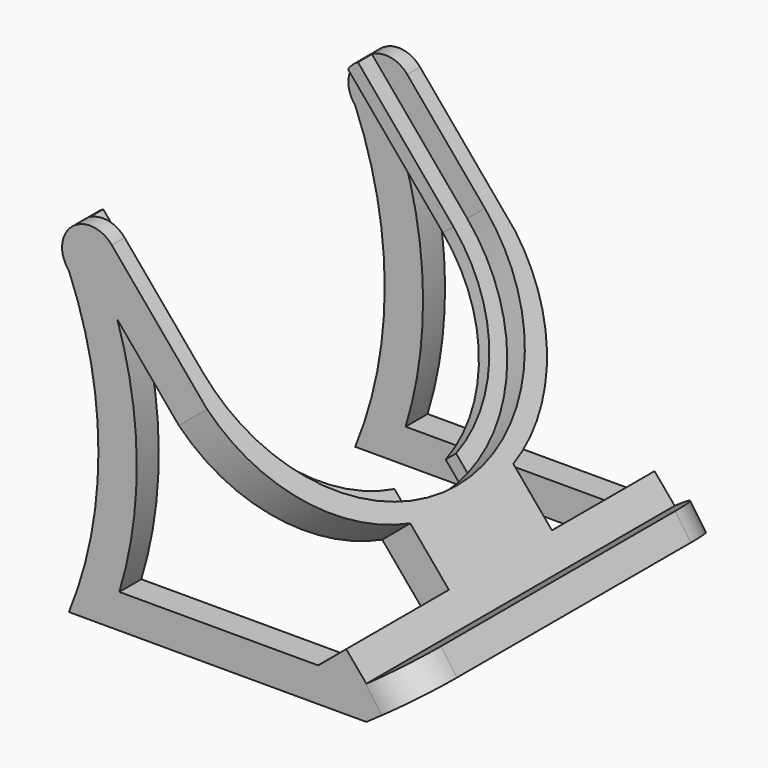
from build123d import *

# Parameters (mm, degrees)
F1_DEPTH  = 53.34
F2_W      = 4.826
F2_H      = 32.1946403572
F3_DEPTH  = 6.35
F5_DEPTH  = 106.68
F7_W      = 91.44
F7_H      = 183.6228075896
F8_DEPTH  = 58.928
F9_DEPTH  = 25.4
F10_R     = 12.8774151417
F11_DEPTH = 10.16
F13_DEPTH = 25.4
F15_DEPTH = 3.81


# Not quite as in the source:
# - a feature names something its author has since deleted; it is built from what else it names


with BuildPart() as f1:
    # F0 (on Front) → F1 (new body, symmetric)
    with BuildSketch(Plane.XZ):
        with BuildLine():
            ThreePointArc((-26.4580316219, 31.2050478526), (-18.2875299748, -10.3937397156), (-26.4580316219, -51.9925272838))
            Line((-26.4580316219, -51.9925272838), (55.8778569108, -51.9925272838))
            Line((55.8778569108, -51.9925272838), (70.650836429, -41.6293909539))
            Line((70.650836429, -41.6293909539), (66.2748063527, -35.3912212887))
            Line((66.2748063527, -35.3912212887), (55.8778569108, -42.6846047493))
            Line((55.8778569108, -42.6846047493), (-14.5902915946, 41.2960643955))
            ThreePointArc((-14.5902915946, 41.2960643955), (-25.6027276184, 42.2233043466), (-26.4580316219, 31.2050478526))
        make_face()
    extrude(amount=F1_DEPTH, both=True)

    # F2 (on face) → F3 (cut)
    with BuildSketch(Plane(origin=(11.772407622, 0, 9.8782228937), x_dir=(0, 1, 0), z_dir=(0.7660444431, 0, 0.6427876097))):
        with BuildLine():
            ThreePointArc((-44.069, 28.7653259742), (-47.673235573, 18.4461288519), (-48.895, 7.584101647))
            Line((-48.895, 7.584101647), (-44.069, 7.584101647))
            Line((-44.069, 7.584101647), (-44.069, 28.7653259742))
        make_face()
        with BuildLine():
            ThreePointArc((44.069, 28.7653259742), (47.673235573, 18.4461288519), (48.895, 7.584101647))
            Line((48.895, 7.584101647), (48.895, 41.0130793115))
            Line((48.895, 41.0130793115), (44.069, 41.0130793115))
            Line((44.069, 41.0130793115), (44.069, 28.7653259742))
        make_face()
        with BuildLine():
            Line((-44.069, 41.0130793115), (-35.6822711903, 41.0130793115))
            ThreePointArc((-35.6822711903, 41.0130793115), (-19.4449371571, 52.4462844288), (0, 56.479101647))
            Line((0, 56.479101647), (0, 73.2077196687))
            Line((0, 73.2077196687), (-44.069, 73.2077196687))
            Line((-44.069, 73.2077196687), (-44.069, 41.0130793115))
        make_face()
        with Locations((-46.482, 57.1103994901)):
            Rectangle(F2_W, F2_H)
        with BuildLine():
            ThreePointArc((0, 56.479101647), (-19.4449371571, 52.4462844288), (-35.6822711903, 41.0130793115))
            Line((-35.6822711903, 41.0130793115), (-28.7155047544, 41.0130793115))
            ThreePointArc((-28.7155047544, 41.0130793115), (-15.3116809054, 48.9075718407), (0, 51.653101647))
            Line((0, 51.653101647), (0, 56.479101647))
        make_face()
        with BuildLine():
            Line((28.7155047544, 41.0130793115), (35.6822711903, 41.0130793115))
            ThreePointArc((35.6822711903, 41.0130793115), (19.4449371571, 52.4462844288), (0, 56.479101647))
            Line((0, 56.479101647), (0, 51.653101647))
            ThreePointArc((0, 51.653101647), (15.3116809054, 48.9075718407), (28.7155047544, 41.0130793115))
        make_face()
        with BuildLine():
            Line((-48.895, 41.0130793115), (-48.895, 7.584101647))
            ThreePointArc((-48.895, 7.584101647), (-47.673235573, 18.4461288519), (-44.069, 28.7653259742))
            Line((-44.069, 28.7653259742), (-44.069, 41.0130793115))
            Line((-44.069, 41.0130793115), (-48.895, 41.0130793115))
        make_face()
        with BuildLine():
            ThreePointArc((0, 56.479101647), (19.4449371571, 52.4462844288), (35.6822711903, 41.0130793115))
            Line((35.6822711903, 41.0130793115), (44.069, 41.0130793115))
            Line((44.069, 41.0130793115), (44.069, 73.082752475))
            Line((44.069, 73.082752475), (0, 73.2077196687))
            Line((0, 73.2077196687), (0, 56.479101647))
        make_face()
        with BuildLine():
            Line((-44.069, 41.0130793115), (-44.069, 28.7653259742))
            ThreePointArc((-44.069, 28.7653259742), (-40.3431305128, 35.2093228303), (-35.6822711903, 41.0130793115))
            Line((-35.6822711903, 41.0130793115), (-44.069, 41.0130793115))
        make_face()
        with BuildLine():
            ThreePointArc((-35.6822711903, 41.0130793115), (-40.3431305128, 35.2093228303), (-44.069, 28.7653259742))
            Line((-44.069, 28.7653259742), (-44.069, 7.584101647))
            ThreePointArc((-44.069, 7.584101647), (-40.0470993957, 25.9772142435), (-28.7155047544, 41.0130793115))
            Line((-28.7155047544, 41.0130793115), (-35.6822711903, 41.0130793115))
        make_face()
        with BuildLine():
            Line((44.069, 7.584101647), (44.069, 28.7653259742))
            ThreePointArc((44.069, 28.7653259742), (40.3431305128, 35.2093228303), (35.6822711903, 41.0130793115))
            Line((35.6822711903, 41.0130793115), (28.7155047544, 41.0130793115))
            ThreePointArc((28.7155047544, 41.0130793115), (40.0470993957, 25.9772142435), (44.069, 7.584101647))
        make_face()
        with BuildLine():
            Line((-44.069, 7.584101647), (-48.895, 7.584101647))
            ThreePointArc((-48.895, 7.584101647), (0, -41.310898353), (48.895, 7.584101647))
            ThreePointArc((48.895, 7.584101647), (47.673235573, 18.4461288519), (44.069, 28.7653259742))
            Line((44.069, 28.7653259742), (44.069, 7.584101647))
            ThreePointArc((44.069, 7.584101647), (0, -36.484898353), (-44.069, 7.584101647))
        make_face()
        with BuildLine():
            Line((0, 7.584101647), (-44.069, 7.584101647))
            ThreePointArc((-44.069, 7.584101647), (0, -36.484898353), (44.069, 7.584101647))
            ThreePointArc((44.069, 7.584101647), (40.0470993957, 25.9772142435), (28.7155047544, 41.0130793115))
            Line((28.7155047544, 41.0130793115), (0, 41.0130793115))
            Line((0, 41.0130793115), (0, 7.584101647))
        make_face()
        with BuildLine():
            ThreePointArc((-28.7155047544, 41.0130793115), (-40.0470993957, 25.9772142435), (-44.069, 7.584101647))
            Line((-44.069, 7.584101647), (0, 7.584101647))
            Line((0, 7.584101647), (0, 41.0130793115))
            Line((0, 41.0130793115), (-28.7155047544, 41.0130793115))
        make_face()
        with BuildLine():
            ThreePointArc((35.6822711903, 41.0130793115), (40.3431305128, 35.2093228303), (44.069, 28.7653259742))
            Line((44.069, 28.7653259742), (44.069, 41.0130793115))
            Line((44.069, 41.0130793115), (35.6822711903, 41.0130793115))
        make_face()
        Polygon((44.069, 41.0130793115), (48.895, 41.0130793115), (48.895, 73.2077196687), (44.069, 73.2077196687), (44.069, 73.082752475), align=None)
    extrude(amount=-F3_DEPTH, mode=Mode.SUBTRACT)

    # F4 (on face) → F5 (cut, through all)
    with BuildSketch(Plane.XZ.offset(53.34)):
        with BuildLine():
            Line((42.5035902841, -42.5519285295), (-13.0547319913, 23.6599016408))
            ThreePointArc((-13.0547319913, 23.6599016408), (-7.6819414216, -9.4041517757), (-12.5113723521, -42.5519285295))
            Line((-12.5113723521, -42.5519285295), (42.5035902841, -42.5519285295))
        make_face()
    extrude(amount=-F5_DEPTH, mode=Mode.SUBTRACT)

    # F7 (on face) → F8 (cut)
    with BuildSketch(Plane(origin=(-41.1275322828, 0, -34.5100971697), x_dir=(0, 1, 0), z_dir=(0.7660444431, 0, 0.6427876097))):
        with Locations((0, -8.2484856248)):
            Rectangle(F7_W, F7_H)
    extrude(amount=F8_DEPTH, mode=Mode.SUBTRACT)

    # F2 (on face) → F9 (cut)
    with BuildSketch(Plane(origin=(11.772407622, 0, 9.8782228937), x_dir=(0, 1, 0), z_dir=(0.7660444431, 0, 0.6427876097))):
        with BuildLine():
            ThreePointArc((-28.7155047544, 41.0130793115), (-40.0470993957, 25.9772142435), (-44.069, 7.584101647))
            Line((-44.069, 7.584101647), (0, 7.584101647))
            Line((0, 7.584101647), (0, 41.0130793115))
            Line((0, 41.0130793115), (-28.7155047544, 41.0130793115))
        make_face()
        with BuildLine():
            Line((0, 7.584101647), (-44.069, 7.584101647))
            ThreePointArc((-44.069, 7.584101647), (0, -36.484898353), (44.069, 7.584101647))
            ThreePointArc((44.069, 7.584101647), (40.0470993957, 25.9772142435), (28.7155047544, 41.0130793115))
            Line((28.7155047544, 41.0130793115), (0, 41.0130793115))
            Line((0, 41.0130793115), (0, 7.584101647))
        make_face()
        with BuildLine():
            ThreePointArc((-35.6822711903, 41.0130793115), (-40.3431305128, 35.2093228303), (-44.069, 28.7653259742))
            Line((-44.069, 28.7653259742), (-44.069, 7.584101647))
            ThreePointArc((-44.069, 7.584101647), (-40.0470993957, 25.9772142435), (-28.7155047544, 41.0130793115))
            Line((-28.7155047544, 41.0130793115), (-35.6822711903, 41.0130793115))
        make_face()
        with BuildLine():
            Line((44.069, 7.584101647), (44.069, 28.7653259742))
            ThreePointArc((44.069, 28.7653259742), (40.3431305128, 35.2093228303), (35.6822711903, 41.0130793115))
            Line((35.6822711903, 41.0130793115), (28.7155047544, 41.0130793115))
            ThreePointArc((28.7155047544, 41.0130793115), (40.0470993957, 25.9772142435), (44.069, 7.584101647))
        make_face()
        with BuildLine():
            Line((28.7155047544, 41.0130793115), (35.6822711903, 41.0130793115))
            ThreePointArc((35.6822711903, 41.0130793115), (19.4449371571, 52.4462844288), (0, 56.479101647))
            Line((0, 56.479101647), (0, 51.653101647))
            ThreePointArc((0, 51.653101647), (15.3116809054, 48.9075718407), (28.7155047544, 41.0130793115))
        make_face()
        with BuildLine():
            ThreePointArc((0, 56.479101647), (-19.4449371571, 52.4462844288), (-35.6822711903, 41.0130793115))
            Line((-35.6822711903, 41.0130793115), (-28.7155047544, 41.0130793115))
            ThreePointArc((-28.7155047544, 41.0130793115), (-15.3116809054, 48.9075718407), (0, 51.653101647))
            Line((0, 51.653101647), (0, 56.479101647))
        make_face()
        with BuildLine():
            Line((-44.069, 41.0130793115), (-35.6822711903, 41.0130793115))
            ThreePointArc((-35.6822711903, 41.0130793115), (-19.4449371571, 52.4462844288), (0, 56.479101647))
            Line((0, 56.479101647), (0, 73.2077196687))
            Line((0, 73.2077196687), (-44.069, 73.2077196687))
            Line((-44.069, 73.2077196687), (-44.069, 41.0130793115))
        make_face()
        with BuildLine():
            Line((-44.069, 41.0130793115), (-44.069, 28.7653259742))
            ThreePointArc((-44.069, 28.7653259742), (-40.3431305128, 35.2093228303), (-35.6822711903, 41.0130793115))
            Line((-35.6822711903, 41.0130793115), (-44.069, 41.0130793115))
        make_face()
        with BuildLine():
            ThreePointArc((0, 56.479101647), (19.4449371571, 52.4462844288), (35.6822711903, 41.0130793115))
            Line((35.6822711903, 41.0130793115), (44.069, 41.0130793115))
            Line((44.069, 41.0130793115), (44.069, 73.082752475))
            Line((44.069, 73.082752475), (0, 73.2077196687))
            Line((0, 73.2077196687), (0, 56.479101647))
        make_face()
        with BuildLine():
            ThreePointArc((35.6822711903, 41.0130793115), (40.3431305128, 35.2093228303), (44.069, 28.7653259742))
            Line((44.069, 28.7653259742), (44.069, 41.0130793115))
            Line((44.069, 41.0130793115), (35.6822711903, 41.0130793115))
        make_face()
        with BuildLine():
            Line((0, 51.653101647), (0, 41.0130793115))
            Line((0, 41.0130793115), (28.7155047544, 41.0130793115))
            ThreePointArc((28.7155047544, 41.0130793115), (15.3116809054, 48.9075718407), (0, 51.653101647))
        make_face()
        with BuildLine():
            ThreePointArc((0, 51.653101647), (-15.3116809054, 48.9075718407), (-28.7155047544, 41.0130793115))
            Line((-28.7155047544, 41.0130793115), (0, 41.0130793115))
            Line((0, 41.0130793115), (0, 51.653101647))
        make_face()
    extrude(amount=-F9_DEPTH, mode=Mode.SUBTRACT)

    # F10
    f10_edges = [f1.edges().sort_by_distance(p)[0] for p in [
        (68.462821, -53.34, -38.510306),
        (68.462821, 53.34, -38.510306),
    ]]
    fillet(f10_edges, radius=F10_R)

    # F2 (on face) → F11 (cut)
    with BuildSketch(Plane(origin=(11.772407622, 0, 9.8782228937), x_dir=(0, 1, 0), z_dir=(0.7660444431, 0, 0.6427876097))):
        with BuildLine():
            ThreePointArc((-17.8272557182, -43.3336769488), (-42.4057040411, -27.2576552243), (-53.34, 0))
            Line((-53.34, 0), (-53.34, -59.9567629397))
            Line((-53.34, -59.9567629397), (-17.8272557182, -59.9567629397))
            Line((-17.8272557182, -59.9567629397), (-17.8272557182, -43.3336769488))
        make_face()
        with BuildLine():
            Line((53.34, -59.9567629397), (53.34, 0))
            ThreePointArc((53.34, 0), (42.4057040411, -27.2576552243), (17.8272557182, -43.3336769488))
            Line((17.8272557182, -43.3336769488), (17.8272557182, -59.9567629397))
            Line((17.8272557182, -59.9567629397), (53.34, -59.9567629397))
        make_face()
    extrude(amount=-F11_DEPTH, mode=Mode.SUBTRACT)

    # F12 (on face) → F13 (cut)
    with BuildSketch(Plane(origin=(6.9080254082, 0, 5.7965215722), x_dir=(0, 1, 0), z_dir=(0.7660444431, 0, 0.6427876097))):
        with BuildLine():
            ThreePointArc((0, -36.484898353), (-5.3721205729, -36.1562353608), (-10.6641114754, -35.1751486673))
            Line((-10.6641114754, -35.1751486673), (-10.6641114754, -40.1337959538))
            ThreePointArc((-10.6641114754, -40.1337959538), (-5.3644394772, -41.0157318311), (0, -41.310898353))
            Line((0, -41.310898353), (0, -36.484898353))
        make_face()
        with BuildLine():
            ThreePointArc((10.6641114754, -35.1751486673), (5.3721205729, -36.1562353608), (0, -36.484898353))
            Line((0, -36.484898353), (0, -41.310898353))
            ThreePointArc((0, -41.310898353), (5.3644394772, -41.0157318311), (10.6641114754, -40.1337959538))
            Line((10.6641114754, -40.1337959538), (10.6641114754, -35.1751486673))
        make_face()
    extrude(amount=-F13_DEPTH, mode=Mode.SUBTRACT)

    # F14 (on face) → F15 (cut)
    with BuildSketch(Plane(origin=(4.0139346614, 0, 3.3680910939), x_dir=(0, -1, 0), z_dir=(-0.7660444431, 0, -0.6427876097))):
        with BuildLine():
            ThreePointArc((10.6641114754, -40.1337959538), (0, -41.310898353), (-10.6641114754, -40.1337959538))
            Line((-10.6641114754, -40.1337959538), (-10.6641114754, -59.9567629397))
            Line((-10.6641114754, -59.9567629397), (10.6641114754, -59.9567629397))
            Line((10.6641114754, -59.9567629397), (10.6641114754, -40.1337959538))
        make_face()
    extrude(amount=-F15_DEPTH, mode=Mode.SUBTRACT)


solid = f1.part
